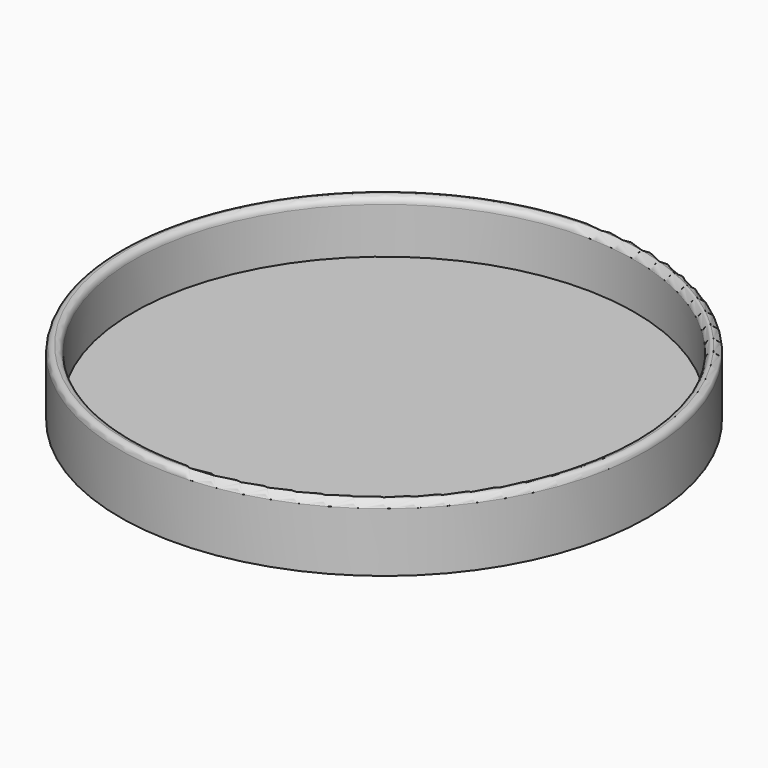
from build123d import *

# Parameters (mm, degrees)
F0_R     = 40.1
F1_DEPTH = 10
F2_R     = 38.1
F3_DEPTH = 8
F4_R     = 0.99999


# Not quite as in the source:
# - a fillet or chamfer is up to 0.001 mm smaller than in the source, because OpenCascade refuses the exact size


with BuildPart() as f1:
    # F0 (on Top) → F1 (new body)
    with BuildSketch(Plane.XY):
        Circle(F0_R)
    extrude(amount=F1_DEPTH)

    # F2 (on face) → F3 (cut)
    with BuildSketch(Plane.XY.offset(10)):
        Circle(F2_R)
    extrude(amount=-F3_DEPTH, mode=Mode.SUBTRACT)

    # F4 (radius 1 in the source; OpenCascade refuses exactly that, so slightly less here)
    f4_edges = [f1.edges().sort_by_distance(p)[0] for p in [
        (-38.1, 0, 10),
        (-40.1, 0, 10),
    ]]
    fillet(f4_edges, radius=F4_R)


solid = f1.part
